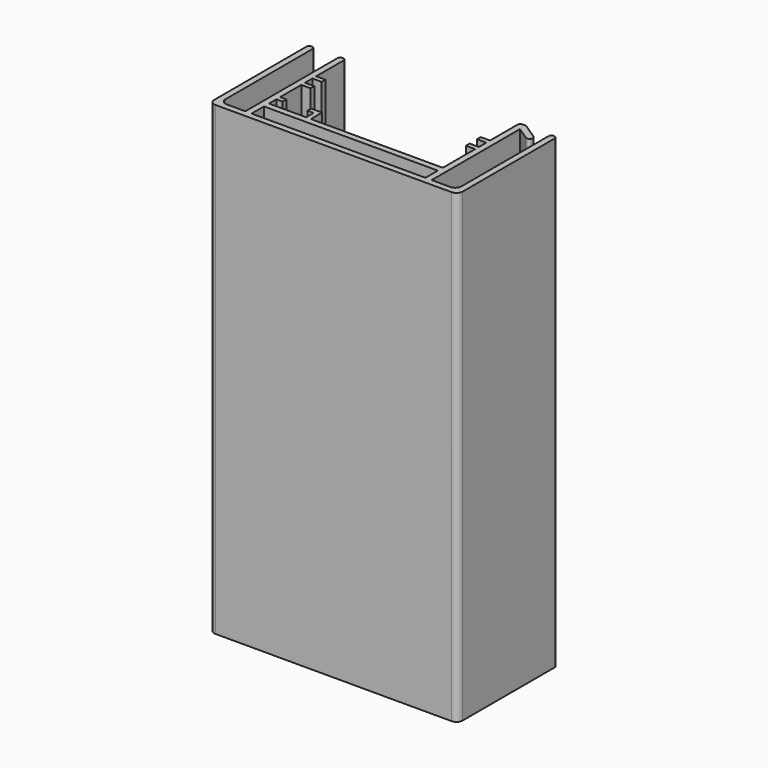
from build123d import *

# Parameters (mm, degrees)
F1_DEPTH = 150
F2_R     = 0.99999


# Not quite as in the source:
# - a fillet or chamfer is up to 0.001 mm smaller than in the source, because OpenCascade refuses the exact size


with BuildPart() as f1:
    # F0 (on Top) → F1 (new body)
    with BuildSketch(Plane.XY):
        Polygon((29.2243703455, 8.5721745163), (29.2243703455, 6.1646732221), (34.1438145412, 2.8682211694), (35.2571452463, 4.5296948349), align=None)
        with BuildLine():
            ThreePointArc((-40.7756296545, -29.4393073201), (-40.1898432169, -30.8535208825), (-38.7756296545, -31.4393073201))
            Line((-38.7756296545, -31.4393073201), (37.2243703455, -31.4393073201))
            ThreePointArc((37.2243703455, -31.4393073201), (38.6385839078, -30.8535208825), (39.2243703455, -29.4393073201))
            Line((39.2243703455, -29.4393073201), (39.2243703455, 8.5606926799))
            Line((39.2243703455, 8.5606926799), (37.2243703455, 8.5606926799))
            Line((37.2243703455, 8.5606926799), (37.2243703455, -27.4393073201))
            ThreePointArc((37.2243703455, -27.4393073201), (36.6385839078, -28.8535208825), (35.2243703455, -29.4393073201))
            Line((35.2243703455, -29.4393073201), (29.2243703455, -29.4393073201))
            Line((29.2243703455, -29.4393073201), (29.2243703455, 6.1646732221))
            Line((29.2243703455, 6.1646732221), (29.2243703455, 8.5721745163))
            Line((29.2243703455, 8.5721745163), (27.2243703455, 8.5721745163))
            Line((27.2243703455, 8.5721745163), (27.2243703455, -3.4278254837))
            Line((27.2243703455, -3.4278254837), (24.2243703455, -3.4278254837))
            Line((24.2243703455, -3.4278254837), (24.2243703455, -4.9278254837))
            Line((24.2243703455, -4.9278254837), (27.2243703455, -4.9278254837))
            Line((27.2243703455, -4.9278254837), (27.2243703455, -7.9278254837))
            Line((27.2243703455, -7.9278254837), (24.2243703455, -7.9278254837))
            Line((24.2243703455, -7.9278254837), (24.2243703455, -9.4278254837))
            Line((24.2243703455, -9.4278254837), (27.2243703455, -9.4278254837))
            Line((27.2243703455, -9.4278254837), (27.2243703455, -22.4393073201))
            Line((27.2243703455, -22.4393073201), (-15.2756296545, -22.4393073201))
            Line((-15.2756296545, -22.4393073201), (-15.2756296545, -17.9393073201))
            Line((-15.2756296545, -17.9393073201), (-18.7756296545, -17.9393073201))
            Line((-18.7756296545, -17.9393073201), (-18.7756296545, -19.4393073201))
            Line((-18.7756296545, -19.4393073201), (-16.7756296545, -19.4393073201))
            Line((-16.7756296545, -19.4393073201), (-16.7756296545, -22.4393073201))
            Line((-16.7756296545, -22.4393073201), (-28.7756296545, -22.4393073201))
            Line((-28.7756296545, -22.4393073201), (-28.7756296545, -19.4393073201))
            Line((-28.7756296545, -19.4393073201), (-26.7756296545, -19.4393073201))
            Line((-26.7756296545, -19.4393073201), (-26.7756296545, -17.9393073201))
            Line((-26.7756296545, -17.9393073201), (-28.7756296545, -17.9393073201))
            Line((-28.7756296545, -17.9393073201), (-28.7756296545, -9.4278254837))
            Line((-28.7756296545, -9.4278254837), (-25.7756296545, -9.4278254837))
            Line((-25.7756296545, -9.4278254837), (-25.7756296545, -7.9278254837))
            Line((-25.7756296545, -7.9278254837), (-28.7756296545, -7.9278254837))
            Line((-28.7756296545, -7.9278254837), (-28.7756296545, -4.9278254837))
            Line((-28.7756296545, -4.9278254837), (-25.7756296545, -4.9278254837))
            Line((-25.7756296545, -4.9278254837), (-25.7756296545, -3.4278254837))
            Line((-25.7756296545, -3.4278254837), (-28.7756296545, -3.4278254837))
            Line((-28.7756296545, -3.4278254837), (-28.7756296545, 8.5721745163))
            Line((-28.7756296545, 8.5721745163), (-30.7756296545, 8.5721745163))
            Line((-30.7756296545, 8.5721745163), (-30.7756296545, -29.4393073201))
            Line((-30.7756296545, -29.4393073201), (-36.7756296545, -29.4393073201))
            ThreePointArc((-36.7756296545, -29.4393073201), (-38.1898432169, -28.8535208825), (-38.7756296545, -27.4393073201))
            Line((-38.7756296545, -27.4393073201), (-38.7756296545, 8.5606926799))
            Line((-38.7756296545, 8.5606926799), (-40.7756296545, 8.5606926799))
            Line((-40.7756296545, 8.5606926799), (-40.7756296545, -29.4393073201))
        make_face()
        Polygon((-28.7756296545, -24.4393073201), (27.2243703455, -24.4393073201), (27.2243703455, -29.4393073201), (-15.2756296545, -29.4393073201), (-16.7756296545, -29.4393073201), (-28.7756296545, -29.4393073201), (-28.7756296545, -26.4393073201), (-28.7756296545, -24.9393073201), align=None, mode=Mode.SUBTRACT)
    extrude(amount=F1_DEPTH)

    # F2 (radius 1 in the source; OpenCascade refuses exactly that, so slightly less here)
    f2_edges = [f1.edges().sort_by_distance(p)[0] for p in [
        (-40.77563, 8.560693, 75),
        (-38.77563, 8.560693, 75),
        (-30.77563, 8.572175, 75),
        (-28.77563, 8.572175, 75),
        (27.22437, 8.572175, 75),
        (29.22437, 8.572175, 75),
        (35.257145, 4.529695, 75),
        (34.143815, 2.868221, 75),
        (37.22437, 8.560693, 75),
        (39.22437, 8.560693, 75),
    ]]
    fillet(f2_edges, radius=F2_R)


solid = f1.part
